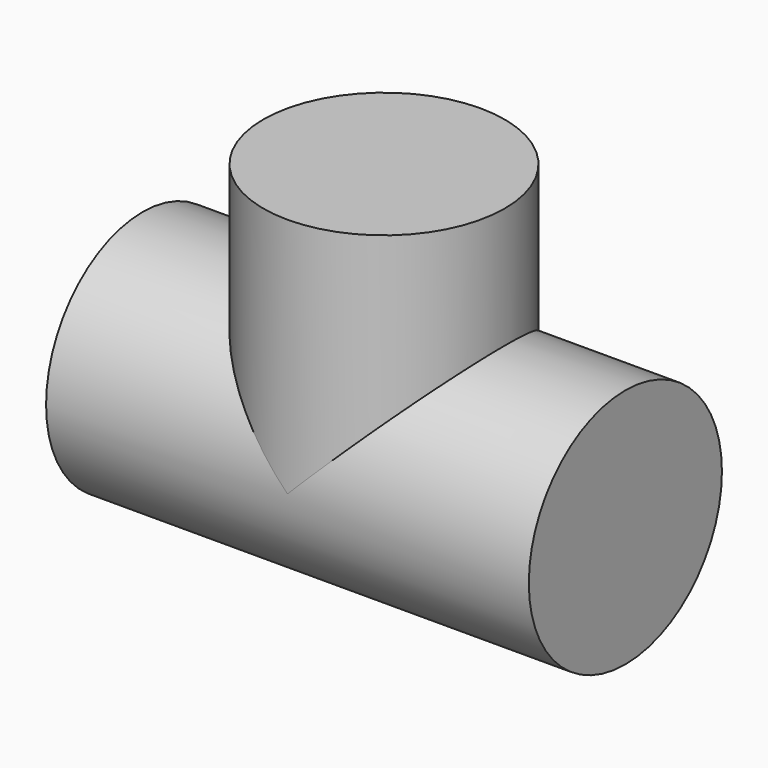
from build123d import *

# Parameters (mm, degrees)
F2_R     = 12.7
F3_DEPTH = 25.4
F5_R     = 12.7
F6_DEPTH = 25.4


# Not quite as in the source:
# - the program builds the solid bodies; features that only make, move or delete a surface that nothing else refers to are left out


with BuildPart() as f3:
    # F2 (on Top) → F3 (new body)
    with BuildSketch(Plane.XY):
        Circle(F2_R)
    extrude(amount=F3_DEPTH)

    # F5 (on Right) → F6 (join, symmetric)
    with BuildSketch(Plane.YZ):
        Circle(F5_R)
    extrude(amount=F6_DEPTH, both=True)


solid = f3.part
